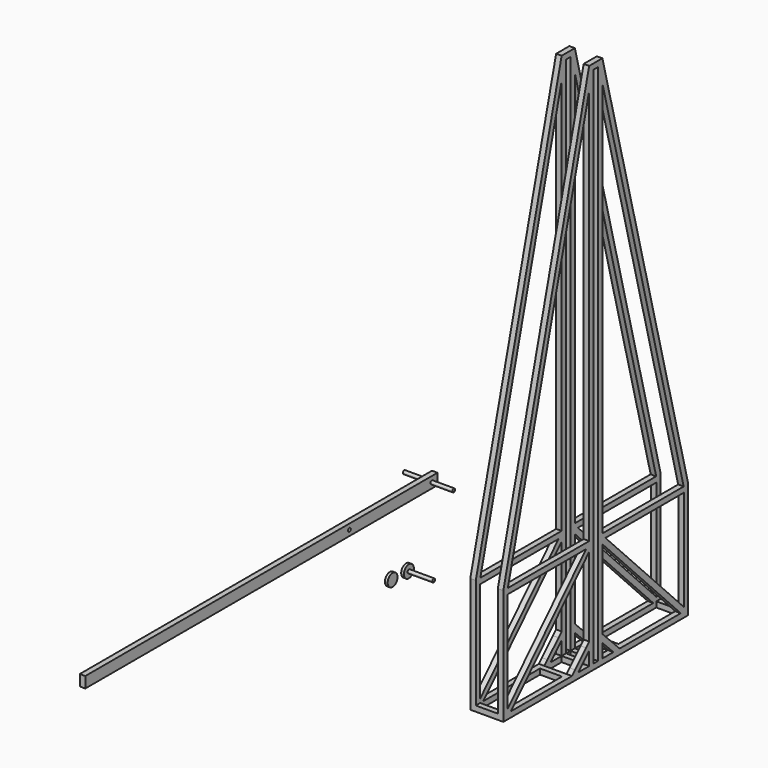
from build123d import *

# Parameters (mm, degrees)
F0_W      = 5.08
F0_H      = 5.08
F1_DEPTH  = 5.08
F4_W      = 5.08
F4_H      = 5.08
F5_DEPTH  = 20.32
F6_W      = 406.4
F6_H      = 10.16
F6_R      = 1.5875
F7_DEPTH  = 5.08
F8_R      = 5.715
F8_R_2    = 1.5875
F9_DEPTH  = 2.54
F10_DEPTH = 25.4
F11_R     = 5.715
F12_DEPTH = 2.54
F15_DEPTH = 25.4
F16_DEPTH = 20.32


# Not quite as in the source:
# - the program builds the solid bodies; features that only make, move or delete a surface that nothing else refers to are left out


with BuildPart() as f1:
    # F0 (on Right) → F1 (new body)
    with BuildSketch(Plane.YZ):
        Polygon((2.54, -101.6), (0, -101.6), (-2.54, -101.6), (-7.62, -101.6), (-20.32, -101.6), (-27.5042048969, -101.6), (-98.0548469748, -101.6), (-101.6, -101.6), (-101.6, -97.9590320281), (-101.6, -5.08), (-101.6, 0), (-106.68, 0), (-106.68, -106.68), (0, -106.68), (106.68, -106.68), (106.68, 0), (101.6, 0), (101.6, -5.08), (101.6, -97.9590320281), (101.6, -101.6), (98.0548469748, -101.6), (27.5042048969, -101.6), (20.32, -101.6), (7.62, -101.6), align=None)
        Polygon((101.4354498343, 0), (7.62, 0), (7.62, -5.08), (11.1651530252, -5.08), (101.6, -5.08), (101.6, 0), align=None)
        Polygon((-7.62, -5.08), (-7.62, 0), (-101.4354498343, 0), (-101.6, 0), (-101.6, -5.08), (-11.1651530252, -5.08), align=None)
        Polygon((2.54, 381), (2.54, 0), (7.62, 0), (7.62, 365.6397019183), (7.62, 381), align=None)
        Polygon((-7.62, 0), (-2.54, 0), (-2.54, 381), (-7.62, 381), (-7.62, 365.6397019183), align=None)
        Polygon((-2.54, 381), (2.54, 381), (7.62, 381), (7.62, 386.08), (-7.62, 386.08), (-7.62, 381), align=None)
        Polygon((-2.54, -101.6), (-2.54, -5.08), (-7.62, -5.08), (-7.62, -8.7209679719), (-7.62, -81.7157951031), (-7.62, -88.9), (-7.62, -101.6), align=None)
        Polygon((-7.62, -8.7209679719), (-7.62, -5.08), (-11.1651530252, -5.08), (-101.6, -97.9590320281), (-101.6, -101.6), (-98.0548469748, -101.6), align=None)
        with Locations((5.08, -2.54)):
            Rectangle(F0_W, F0_H)
        with Locations((-5.08, -2.54)):
            Rectangle(F0_W, F0_H)
        Polygon((7.62, -5.08), (2.54, -5.08), (2.54, -101.6), (7.62, -101.6), (7.62, -88.9), (7.62, -81.7157951031), (7.62, -8.7209679719), align=None)
        Polygon((11.1651530252, -5.08), (7.62, -5.08), (7.62, -8.7209679719), (98.0548469748, -101.6), (101.6, -101.6), (101.6, -97.9590320281), align=None)
        Polygon((11.2121024484, -85.3078975516), (7.62, -81.7157951031), (7.62, -88.9), (20.32, -101.6), (27.5042048969, -101.6), (23.9121024484, -98.0078975516), align=None)
        Polygon((-27.5042048969, -101.6), (-20.32, -101.6), (-7.62, -88.9), (-7.62, -81.7157951031), (-11.2121024484, -85.3078975516), (-23.9121024484, -98.0078975516), align=None)
        Polygon((7.62, 365.6397019183), (101.4354498343, 0), (101.6, 0), (106.68, 0), (7.62, 386.08), (7.62, 381), align=None)
        Polygon((-101.6, 0), (-101.4354498343, 0), (-7.62, 365.6397019183), (-7.62, 381), (-7.62, 386.08), (-106.68, 0), align=None)
    extrude(amount=F1_DEPTH)


with BuildPart() as f2_1:
    # F2: copy of F1
    add(f1.part)


with BuildPart() as f2_1_1:
    # F3: moved
    add(f2_1.part.moved(Location((-25.4, 0, 0))))


with BuildPart() as f1_1:
    add(f1.part)

    add(f2_1_1.part)  # F5 merges F2_1
    # F4 (on face) → F5 (join, through all)
    with BuildSketch(Plane(origin=(0, 0, 0), x_dir=(0, -1, 0), z_dir=(-1, 0, 0))):
        with Locations((-104.14, -104.14)):
            Rectangle(F4_W, F4_H)
        with Locations((-30.0442048969, -104.14)):
            Rectangle(F4_W, F4_H)
        with Locations((-5.08, -104.14)):
            Rectangle(F4_W, F4_H)
        with Locations((5.08, -104.14)):
            Rectangle(F4_W, F4_H)
        with Locations((30.0442048969, -104.14)):
            Rectangle(F4_W, F4_H)
        with Locations((104.14, -104.14)):
            Rectangle(F4_W, F4_H)
    extrude(amount=F5_DEPTH)


with BuildPart() as f7:
    # F6 (on Right) → F7 (new body)
    with BuildSketch(Plane.YZ):
        with Locations((-385.7845490456, 121.5760712194)):
            Rectangle(F6_W, F6_H)
        with Locations((-284.1845490456, 121.5760712194)):
            Circle(F6_R, mode=Mode.SUBTRACT)
        with BuildLine():
            ThreePointArc((-190.8395490456, 121.5760712194), (-189.2520490456, 123.1635712194), (-187.6645490456, 121.5760712194))
            ThreePointArc((-187.6645490456, 121.5760712194), (-189.2520490456, 119.9885712194), (-190.8395490456, 121.5760712194))
        make_face(mode=Mode.SUBTRACT)
        with BuildLine():
            ThreePointArc((-190.8395490456, 121.5760712194), (-189.2520490456, 119.9885712194), (-187.6645490456, 121.5760712194))
            Line((-187.6645490456, 121.5760712194), (-190.8395490456, 121.5760712194))
        make_face()
        with BuildLine():
            Line((-190.8395490456, 121.5760712194), (-187.6645490456, 121.5760712194))
            ThreePointArc((-187.6645490456, 121.5760712194), (-189.2520490456, 123.1635712194), (-190.8395490456, 121.5760712194))
        make_face()
    extrude(amount=F7_DEPTH)

    # F6 (on Right) → F15 (join)
    with BuildSketch(Plane.YZ):
        with BuildLine():
            Line((-190.8395490456, 121.5760712194), (-187.6645490456, 121.5760712194))
            ThreePointArc((-187.6645490456, 121.5760712194), (-189.2520490456, 123.1635712194), (-190.8395490456, 121.5760712194))
        make_face()
        with BuildLine():
            ThreePointArc((-190.8395490456, 121.5760712194), (-189.2520490456, 119.9885712194), (-187.6645490456, 121.5760712194))
            Line((-187.6645490456, 121.5760712194), (-190.8395490456, 121.5760712194))
        make_face()
    extrude(amount=F15_DEPTH)

    # F6 (on Right) → F16 (join)
    with BuildSketch(Plane.YZ):
        with BuildLine():
            Line((-190.8395490456, 121.5760712194), (-187.6645490456, 121.5760712194))
            ThreePointArc((-187.6645490456, 121.5760712194), (-189.2520490456, 123.1635712194), (-190.8395490456, 121.5760712194))
        make_face()
        with BuildLine():
            ThreePointArc((-190.8395490456, 121.5760712194), (-189.2520490456, 119.9885712194), (-187.6645490456, 121.5760712194))
            Line((-187.6645490456, 121.5760712194), (-190.8395490456, 121.5760712194))
        make_face()
    extrude(amount=-F16_DEPTH)


with BuildPart() as f9:
    # F8 (on Right) → F9 (new body)
    with BuildSketch(Plane.YZ):
        with Locations((-212.4280929565, 57.8589513898)):
            Circle(F8_R)
        with Locations((-212.4280929565, 57.8589513898)):
            Circle(F8_R_2, mode=Mode.SUBTRACT)
        with Locations((-212.4280929565, 57.8589513898)):
            Circle(F8_R_2)
    extrude(amount=F9_DEPTH)

    # F8 (on Right) → F10 (join)
    with BuildSketch(Plane.YZ):
        with Locations((-212.4280929565, 57.8589513898)):
            Circle(F8_R_2)
    extrude(amount=F10_DEPTH)


with BuildPart() as f12:
    # F11 (on Right) → F12 (new body)
    with BuildSketch(Plane.YZ):
        with Locations((-231.2091737986, 58.4822148085)):
            Circle(F11_R)
    extrude(amount=F12_DEPTH)


solid = Compound([f1_1.part, f7.part, f9.part, f12.part])
